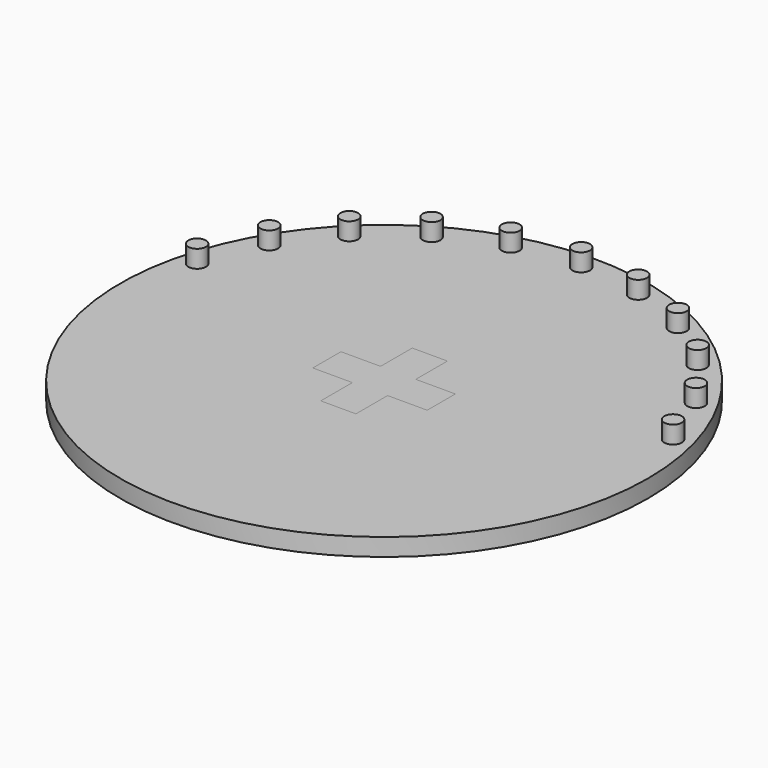
from build123d import *

# Parameters (mm, degrees)
F0_R     = 300
F0_R_2   = 10
F0_R_3   = 20
F1_DEPTH = 20
F2_R     = 10
F3_DEPTH = 20
F5_DEPTH = 10
F7_DEPTH = 10
F8_R     = 20
F9_DEPTH = 80


with BuildPart() as f1:
    # F0 (on Top) → F1 (new body)
    with BuildSketch(Plane.XY):
        Circle(F0_R)
        with Locations((-270.4592313609, 72.4693326287)):
            Circle(F0_R_2, mode=Mode.SUBTRACT)
        with Locations((-242.4871130596, 140)):
            Circle(F0_R_2, mode=Mode.SUBTRACT)
        with Locations((-197.9898987322, 197.9898987322)):
            Circle(F0_R_2, mode=Mode.SUBTRACT)
        with Locations((-140, 242.4871130596)):
            Circle(F0_R_2, mode=Mode.SUBTRACT)
        with Locations((-72.4693326287, 270.4592313609)):
            Circle(F0_R_2, mode=Mode.SUBTRACT)
        Circle(F0_R_3, mode=Mode.SUBTRACT)
        with Locations((270.4592313609, 72.4693326287)):
            Circle(F0_R_2, mode=Mode.SUBTRACT)
        with Locations((242.4871130596, 140)):
            Circle(F0_R_2, mode=Mode.SUBTRACT)
        with Locations((0, 280)):
            Circle(F0_R_2, mode=Mode.SUBTRACT)
        with Locations((72.4693326287, 270.4592313609)):
            Circle(F0_R_2, mode=Mode.SUBTRACT)
        with Locations((140, 242.4871130596)):
            Circle(F0_R_2, mode=Mode.SUBTRACT)
        with Locations((197.9898987322, 197.9898987322)):
            Circle(F0_R_2, mode=Mode.SUBTRACT)
    extrude(amount=F1_DEPTH)

    # F4 (on face) → F5 (cut)
    with BuildSketch(Plane.XY.offset(20)):
        Polygon((-65, 20), (-65, 0), (-65, -20), (-20, -20), (-20, -65), (0, -65), (20, -65), (20, -20), (65, -20), (65, 0), (65, 20), (20, 20), (20, 65), (0, 65), (-20, 65), (-20, 20), align=None)
    extrude(amount=-F5_DEPTH, mode=Mode.SUBTRACT)


with BuildPart() as f3:
    # F2 (on face) → F3 (new body, symmetric)
    with BuildSketch(Plane.XY.offset(20)):
        with Locations((-270.4592313609, 72.4693326287)):
            Circle(F2_R)
    extrude(amount=F3_DEPTH, both=True)


with BuildPart() as f3b:
    # F2 (on face) → F3, piece 2 (new body, symmetric)
    with BuildSketch(Plane.XY.offset(20)):
        with Locations((-242.4871130596, 140)):
            Circle(F2_R)
    extrude(amount=F3_DEPTH, both=True)


with BuildPart() as f3c:
    # F2 (on face) → F3, piece 3 (new body, symmetric)
    with BuildSketch(Plane.XY.offset(20)):
        with Locations((-197.9898987322, 197.9898987322)):
            Circle(F2_R)
    extrude(amount=F3_DEPTH, both=True)


with BuildPart() as f3d:
    # F2 (on face) → F3, piece 4 (new body, symmetric)
    with BuildSketch(Plane.XY.offset(20)):
        with Locations((-140, 242.4871130596)):
            Circle(F2_R)
    extrude(amount=F3_DEPTH, both=True)


with BuildPart() as f3e:
    # F2 (on face) → F3, piece 5 (new body, symmetric)
    with BuildSketch(Plane.XY.offset(20)):
        with Locations((-72.4693326287, 270.4592313609)):
            Circle(F2_R)
    extrude(amount=F3_DEPTH, both=True)


with BuildPart() as f3f:
    # F2 (on face) → F3, piece 6 (new body, symmetric)
    with BuildSketch(Plane.XY.offset(20)):
        with Locations((0, 280)):
            Circle(F2_R)
    extrude(amount=F3_DEPTH, both=True)


with BuildPart() as f3g:
    # F2 (on face) → F3, piece 7 (new body, symmetric)
    with BuildSketch(Plane.XY.offset(20)):
        with Locations((270.4592313609, 72.4693326287)):
            Circle(F2_R)
    extrude(amount=F3_DEPTH, both=True)


with BuildPart() as f3h:
    # F2 (on face) → F3, piece 8 (new body, symmetric)
    with BuildSketch(Plane.XY.offset(20)):
        with Locations((242.4871130596, 140)):
            Circle(F2_R)
    extrude(amount=F3_DEPTH, both=True)


with BuildPart() as f3i:
    # F2 (on face) → F3, piece 9 (new body, symmetric)
    with BuildSketch(Plane.XY.offset(20)):
        with Locations((197.9898987322, 197.9898987322)):
            Circle(F2_R)
    extrude(amount=F3_DEPTH, both=True)


with BuildPart() as f3j:
    # F2 (on face) → F3, piece 10 (new body, symmetric)
    with BuildSketch(Plane.XY.offset(20)):
        with Locations((140, 242.4871130596)):
            Circle(F2_R)
    extrude(amount=F3_DEPTH, both=True)


with BuildPart() as f3k:
    # F2 (on face) → F3, piece 11 (new body, symmetric)
    with BuildSketch(Plane.XY.offset(20)):
        with Locations((72.4693326287, 270.4592313609)):
            Circle(F2_R)
    extrude(amount=F3_DEPTH, both=True)


with BuildPart() as f7:
    # F6 (on face) → F7 (new body)
    with BuildSketch(Plane.XY.offset(20)):
        Polygon((-65, 20), (-65, -20), (-20, -20), (-20, -65), (20, -65), (20, -20), (65, -20), (65, 20), (20, 20), (20, 65), (-20, 65), (-20, 20), align=None)
    extrude(amount=-F7_DEPTH)

    # F8 (on face) → F9 (join)
    with BuildSketch(Plane(origin=(0, 0, 10), x_dir=(1, 0, 0), z_dir=(0, 0, -1))):
        Circle(F8_R)
    extrude(amount=F9_DEPTH)


solid = Compound([f1.part, f3.part, f3b.part, f3c.part, f3d.part, f3e.part, f3f.part, f3g.part, f3h.part, f3i.part, f3j.part, f3k.part, f7.part])
